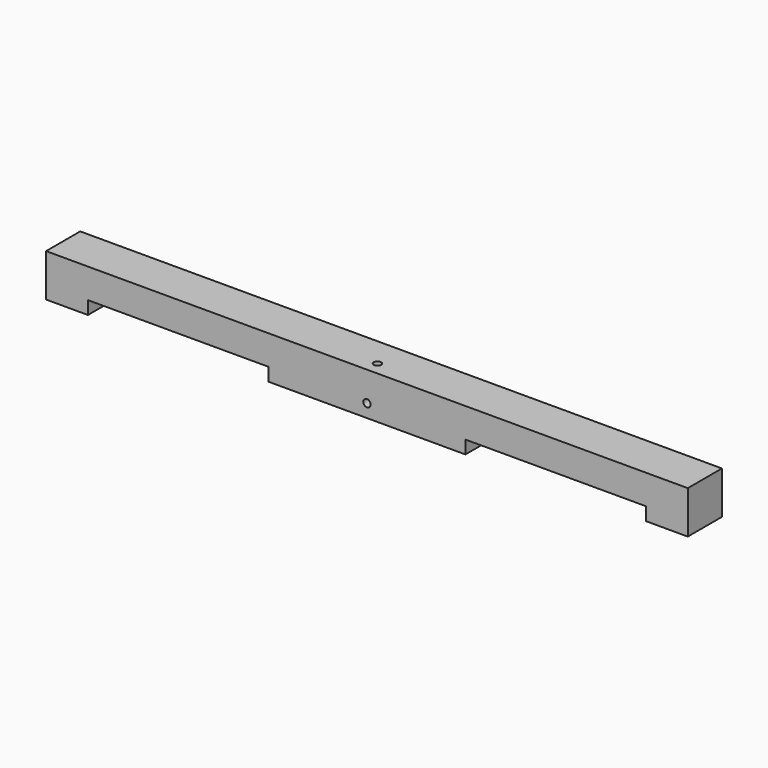
from build123d import *

# Parameters (mm, degrees)
F0_W     = 26
F0_H     = 26
F1_DEPTH = 195.5
F3_W     = 110
F3_H     = 8
F4_DEPTH = 26
F6_D     = 4.5
F8_D     = 4.5


# Not quite as in the source:
# - a pattern or mirror of a feature is missing from the dataset's text; its kind, count and spacing are read off the source's solid


with BuildPart() as f1:
    # F0 (on Right) → F1 (new body, symmetric)
    with BuildSketch(Plane.YZ):
        with Locations((0, 13)):
            Rectangle(F0_W, F0_H)
    extrude(amount=F1_DEPTH, both=True)

    # F3 (on face) → F4 (cut, through all)
    with BuildSketch(Plane.XZ.offset(13)):
        with Locations((-115, 4)):
            Rectangle(F3_W, F3_H)
    f4 = extrude(amount=-F4_DEPTH, mode=Mode.SUBTRACT)

    # F4_copies: F4 across plane
    add(f4.mirror(Plane(origin=(0, 0, 0), x_dir=(0, 0, 1), z_dir=(1, 0, 0))), mode=Mode.SUBTRACT)

    # F6 (through all)
    with Locations(Plane.XZ.offset(13)):
        with Locations((0, 8)):
            Hole(F6_D / 2)

    # F8 (through all)
    with Locations(Plane.XY.offset(26)):
        with Locations((0, -5)):
            Hole(F8_D / 2)


solid = f1.part
